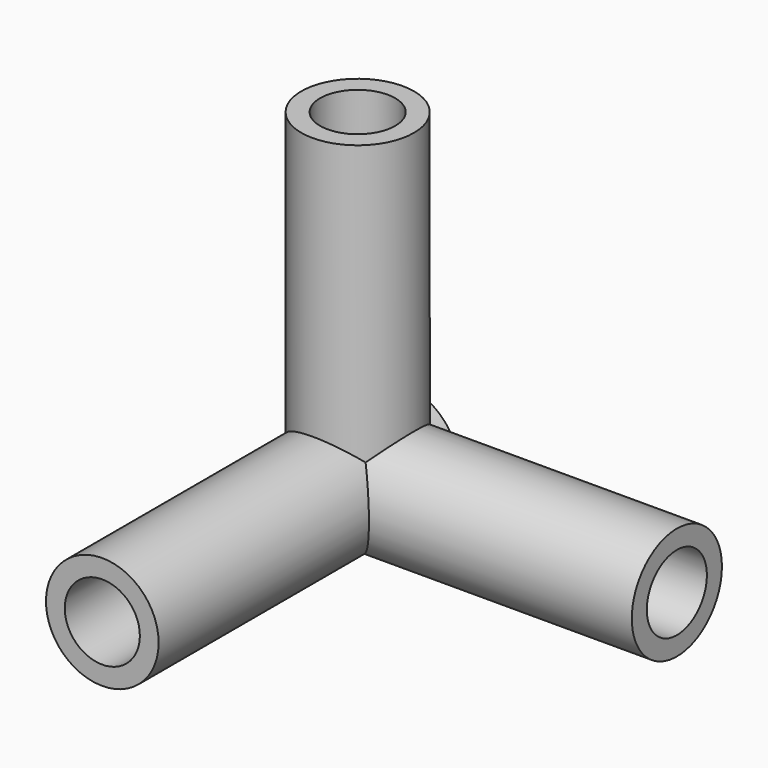
from build123d import *
from build123d import SkipClean  # not in build123d's __all__

# Parameters (mm, degrees)
F2_R      = 15
F3_DEPTH  = 100
F4_R      = 10
F5_DEPTH  = 25
F6_R      = 15
F7_DEPTH  = 85
F8_R      = 10
F9_DEPTH  = 25
F10_R     = 15
F11_DEPTH = 85
F12_R     = 10
F13_DEPTH = 25


with BuildPart() as f3:
    # F2 (on Front) → F3 (new body)
    with BuildSketch(Plane.XZ):
        Circle(F2_R)
    extrude(amount=F3_DEPTH)

    # F4 (on face) → F5 (cut)
    with BuildSketch(Plane.XZ.offset(100)):
        Circle(F4_R)
    extrude(amount=-F5_DEPTH, mode=Mode.SUBTRACT)

    # F6 (on Top) → F7 (join)
    with BuildSketch(Plane.XY):
        with Locations((0, -15)):
            Circle(F6_R)
    with SkipClean():  # cleaning this boolean's faces spoils the solid; the shape is the same uncleaned
        extrude(amount=F7_DEPTH)

    # F8 (on face) → F9 (cut)
    with BuildSketch(Plane.XY.offset(85)):
        with Locations((0, -15)):
            Circle(F8_R)
    with SkipClean():  # cleaning this boolean's faces spoils the solid; the shape is the same uncleaned
        extrude(amount=-F9_DEPTH, mode=Mode.SUBTRACT)

    # F10 (on Right) → F11 (join)
    with BuildSketch(Plane.YZ):
        with Locations((-15, 0)):
            Circle(F10_R)
    extrude(amount=F11_DEPTH)

    # F12 (on face) → F13 (cut)
    with BuildSketch(Plane.YZ.offset(85)):
        with Locations((-15, 0)):
            Circle(F12_R)
    extrude(amount=-F13_DEPTH, mode=Mode.SUBTRACT)


solid = f3.part
